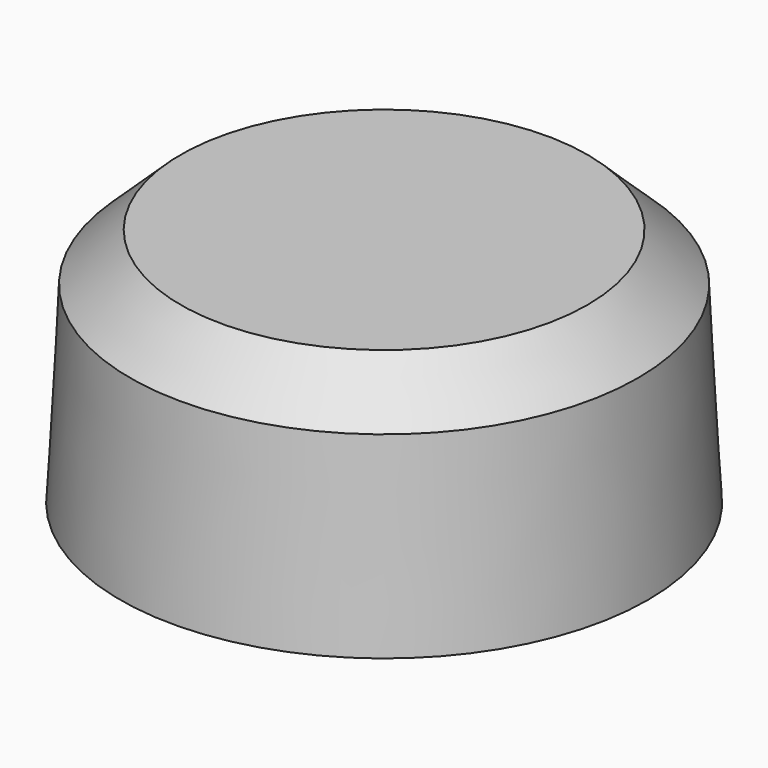
from build123d import *

# Parameters (mm, degrees)
F0_R     = 27.5
F1_DEPTH = 25
F1_TAPER = 3


# Not quite as in the source:
# - a fillet or chamfer that OpenCascade refuses, or shapes differently, is made with other operations: its cross-section is extruded or revolved along the edge and cut away or added


with BuildPart() as f1:
    # F0 (on Top) → F1 (new body)
    with BuildSketch(Plane.XY):
        Circle(F0_R)
    extrude(amount=F1_DEPTH, taper=F1_TAPER)

    # F2: chamfer of 5 on 1 edges, made by hand

    # F2_s1 → F2_t2 (revolve, cut)
    with BuildSketch(Plane.XZ):
        Polygon((26.4514852991, 20.0068523262), (21.1898055179, 25), (26.1898055179, 25), align=None)
    revolve(axis=Axis((0, 0, 25), (0, 0, -1)), mode=Mode.SUBTRACT)


solid = f1.part
